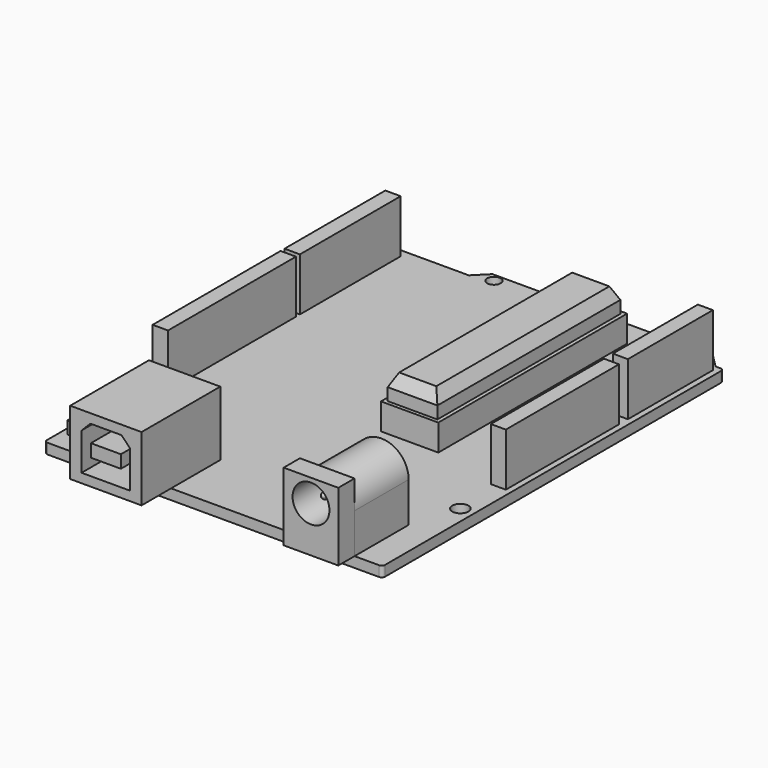
from build123d import *

# Parameters (mm, degrees)
F1_DEPTH   = 1.69
F2_W       = 2.434945175
F2_H       = 23
F3_DEPTH   = 8.6
F2_H_2     = 17.2737486292
F2_W_2     = 2.5
F2_H_3     = 20.481327492
F2_H_4     = 26
F6_DEPTH   = 11
F7_W       = 8.87868274
F7_H       = 11.1249446636
F8_DEPTH   = 3.3
F9_R       = 3
F10_DEPTH  = 12.8
F11_R      = 0.5
F12_DEPTH  = 10
F13_W      = 11.6
F13_H      = 10
F14_DEPTH  = 10.5
F15_W      = 11.6
F15_H      = 10.5
F16_DEPTH  = 6
F18_DEPTH  = 14.14393
F19_W      = 4.8785965383
F19_H      = 2.0820805803
F20_DEPTH  = 14.14393
F21_W      = 6.5
F21_H      = 6.5
F22_DEPTH  = 2
F23_R      = 2.2427667378
F24_DEPTH  = 1
F25_W      = 9.3276520822
F25_H      = 38.3693373368
F26_DEPTH  = 4.29568
F27_W      = 8.0811752376
F27_H      = 37.1907090231
F28_DEPTH  = 2
F30_W      = 6.0478351079
F30_H      = 35.1617564447
F28_FACE_W = 8.0811752376
F28_FACE_H = 37.1907090231
F32_R      = 1.1
F33_DEPTH  = 1.691
F34_R      = 1.1
F34_R_2    = 1.3134018391
F35_DEPTH  = 1.691
F37_ANGLE  = 180


with BuildPart() as f1:
    # F0 (on Top) → F1 (new body)
    with BuildSketch(Plane.XY):
        with BuildLine():
            Line((24.0339115262, 35.744994029), (-11.8138234477, 35.744994029))
            Line((-11.8138234477, 35.744994029), (-13.952996046, 33.6058214307))
            Line((-13.952996046, 33.6058214307), (-25.4879149359, 33.6058214307))
            Line((-25.4879149359, 33.6058214307), (-27.4785661542, 31.6151702124))
            Line((-27.4785661542, 31.6151702124), (-27.4785661542, -35.2069868512))
            ThreePointArc((-27.4785661542, -35.2069868512), (-27.3209875002, -35.5874153749), (-26.9405589764, -35.744994029))
            Line((-26.9405589764, -35.744994029), (26.9657578724, -35.744994029))
            ThreePointArc((26.9657578724, -35.744994029), (27.3283680859, -35.5947959607), (27.4785661542, -35.2321857471))
            Line((27.4785661542, -35.2321857471), (27.4785661542, 33.0678142529))
            ThreePointArc((27.4785661542, 33.0678142529), (27.3209875002, 33.4482427766), (26.9405589764, 33.6058214307))
            Line((26.9405589764, 33.6058214307), (26.1730841245, 33.6058214307))
            Line((26.1730841245, 33.6058214307), (24.0339115262, 35.744994029))
        make_face()
    extrude(amount=F1_DEPTH)

    # F32 (on face) → F33 (cut, through all)
    with BuildSketch(Plane.XY.offset(1.69)):
        with Locations((-10.5248941109, 34.4266854227)):
            Circle(F32_R)
        with Locations((22.7033495903, 34.4266854227)):
            Circle(F32_R)
    extrude(amount=-F33_DEPTH, mode=Mode.SUBTRACT)

    # F34 (on face) → F35 (cut, through all)
    with BuildSketch(Plane.XY.offset(1.69)):
        with Locations((-25.2349545183, -17.141347751)):
            Circle(F34_R)
        with Locations((25.2761915326, -17.141347751)):
            Circle(F34_R_2)
    extrude(amount=-F35_DEPTH, mode=Mode.SUBTRACT)


with BuildPart() as f3:
    # F2 (on face) → F3 (new body)
    with BuildSketch(Plane.XY.offset(1.69)):
        with Locations((25.316230242, 2.0224055983)):
            Rectangle(F2_W, F2_H)
    extrude(amount=F3_DEPTH)


with BuildPart() as f3b:
    # F2 (on face) → F3, piece 2 (new body)
    with BuildSketch(Plane.XY.offset(1.69)):
        with Locations((25.316230242, 23.9592799129)):
            Rectangle(F2_W, F2_H_2)
    extrude(amount=F3_DEPTH)


with BuildPart() as f3c:
    # F2 (on face) → F3, piece 3 (new body)
    with BuildSketch(Plane.XY.offset(1.69)):
        with Locations((-25.2285661542, 22.0511595675)):
            Rectangle(F2_W_2, F2_H_3)
    extrude(amount=F3_DEPTH)


with BuildPart() as f3d:
    # F2 (on face) → F3, piece 4 (new body)
    with BuildSketch(Plane.XY.offset(1.69)):
        with Locations((-25.2285661542, -1.9895041785)):
            Rectangle(F2_W_2, F2_H_4)
    extrude(amount=F3_DEPTH)


with BuildPart() as f6:
    # F5 (on offset) → F6 (new body)
    with BuildSketch(Plane.XZ.offset(35.744994029)):
        with BuildLine():
            Line((14.0722493033, 1.6842637178), (22.9522493033, 1.6842637178))
            Line((22.9522493033, 1.6842637178), (22.9522493033, 8.1842637178))
            ThreePointArc((22.9522493033, 8.1842637178), (18.5122493033, 12.6242637178), (14.0722493033, 8.1842637178))
            Line((14.0722493033, 8.1842637178), (14.0722493033, 1.6842637178))
        make_face()
    extrude(amount=-F6_DEPTH)

    # F7 (on offset) → F8 (join)
    with BuildSketch(Plane.XZ.offset(35.744994029)):
        with Locations((18.5108794831, 7.2514217463)):
            Rectangle(F7_W, F7_H)
    extrude(amount=F8_DEPTH)

    # F9 (on face) → F10 (cut)
    with BuildSketch(Plane.XZ.offset(39.044994029)):
        with Locations((18.5108794831, 9.124157019)):
            Circle(F9_R)
    extrude(amount=-F10_DEPTH, mode=Mode.SUBTRACT)


with BuildPart() as f12:
    # F11 (on face) → F12 (new body)
    with BuildSketch(Plane.XZ.offset(26.244994029)):
        with Locations((18.5108794831, 9.124157019)):
            Circle(F11_R)
    extrude(amount=F12_DEPTH)

    # F36 (on face) → F37 (revolve)
    with BuildSketch(Plane.XZ.offset(36.244994029)):
        with BuildLine():
            ThreePointArc((19.0108794831, 9.124157019), (18.8644328737, 9.4777104096), (18.5108794831, 9.624157019))
            Line((18.5108794831, 9.624157019), (18.5108794831, 8.624157019))
            ThreePointArc((18.5108794831, 8.624157019), (18.8644328737, 8.7706036284), (19.0108794831, 9.124157019))
        make_face()
    revolve(axis=Axis((18.5108794831, -36.244994029, 9.124157019), (0, 0, -1)), revolution_arc=F37_ANGLE)


with BuildPart() as f14:
    # F13 (on face) → F14 (new body)
    with BuildSketch(Plane.XY.offset(1.69)):
        with Locations((-12.6785661542, -30.744994029)):
            Rectangle(F13_W, F13_H)
    extrude(amount=F14_DEPTH)

    # F15 (on face) → F16 (join)
    with BuildSketch(Plane.XZ.offset(35.744994029)):
        with Locations((-12.6785661542, 6.94)):
            Rectangle(F15_W, F15_H)
    extrude(amount=F16_DEPTH)

    # F17 (on face) → F18 (cut)
    with BuildSketch(Plane.XZ.offset(41.744994029)):
        Polygon((-16.6285661542, 9.2491237447), (-16.6285661542, 3.19), (-8.7285661542, 3.19), (-8.7285661542, 9.2515923473), (-10.1669738069, 10.69), (-15.1876898989, 10.69), align=None)
    extrude(amount=-F18_DEPTH, mode=Mode.SUBTRACT)


with BuildPart() as f20:
    # F19 (on face) → F20 (new body, through all)
    with BuildSketch(Plane.XZ.offset(27.601064029)):
        with Locations((-12.6773318529, 6.8805450574)):
            Rectangle(F19_W, F19_H)
    extrude(amount=F20_DEPTH)


with BuildPart() as f22:
    # F21 (on face) → F22 (new body)
    with BuildSketch(Plane.XY.offset(1.69)):
        with Locations((-23.1851451099, -29.143884778)):
            Rectangle(F21_W, F21_H)
    extrude(amount=F22_DEPTH)


with BuildPart() as f24:
    # F23 (on face) → F24 (new body)
    with BuildSketch(Plane.XY.offset(3.69)):
        with Locations((-23.1851451099, -29.143884778)):
            Circle(F23_R)
    extrude(amount=F24_DEPTH)


with BuildPart() as f26:
    # F25 (on face) → F26 (new body)
    with BuildSketch(Plane.XY.offset(1.69)):
        with Locations((8.8037233053, 12.316826851)):
            Rectangle(F25_W, F25_H)
    extrude(amount=F26_DEPTH)


with BuildPart() as f28:
    # F27 (on face) → F28 (new body)
    with BuildSketch(Plane.XY.offset(5.98568)):
        with Locations((8.8037233053, 12.316826851)):
            Rectangle(F27_W, F27_H)
    extrude(amount=F28_DEPTH)


with BuildPart() as f31:
    # F30 (on offset) → F31 section 0
    with BuildSketch(Plane.XY.offset(9.98568)):
        with Locations((8.8047666941, 12.3632361647)):
            Rectangle(F30_W, F30_H)
    # F28_face (on face) → F31 section 1
    with BuildSketch(Plane(origin=(8.8037233053, 12.316826851, 7.98568), x_dir=(1, 0, 0), z_dir=(0, 0, 1))):
        Rectangle(F28_FACE_W, F28_FACE_H)
    loft()


solid = Compound([f1.part, f3.part, f3b.part, f3c.part, f3d.part, f6.part, f12.part, f14.part, f20.part, f22.part, f24.part, f26.part, f28.part, f31.part])
